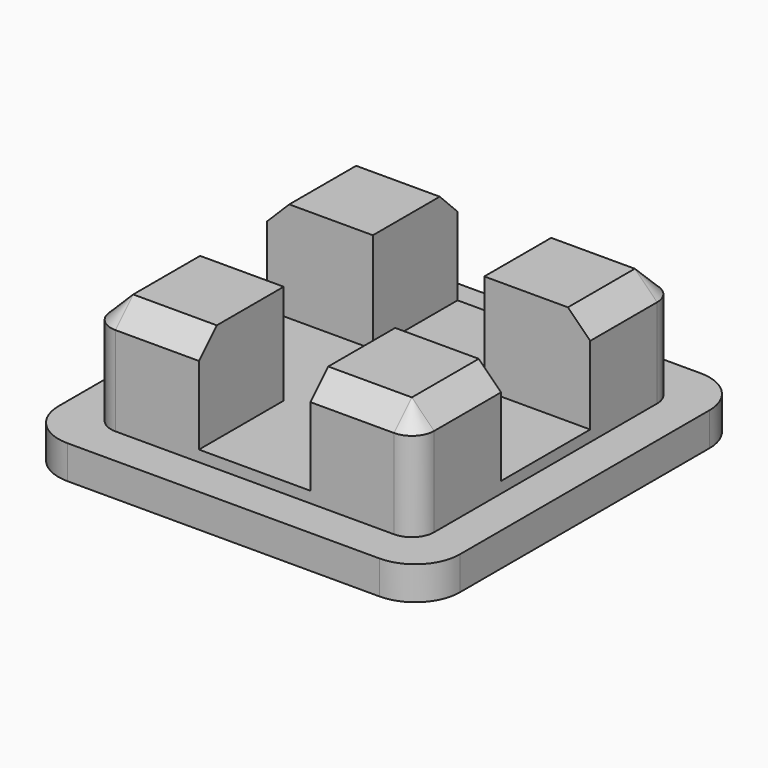
from build123d import *

# Parameters (mm, degrees)
F1_DEPTH = 3
F3_DEPTH = 10
F5_DEPTH = 9
F6_SIZE  = 1.99999


# Not quite as in the source:
# - a fillet or chamfer is up to 0.001 mm smaller than in the source, because OpenCascade refuses the exact size


with BuildPart() as f1:
    # F0 (on Top) → F1 (new body)
    with BuildSketch(Plane.XY):
        with BuildLine():
            Line((16.3916659281, 18.4843443355), (-11.6083340719, 18.4843443355))
            ThreePointArc((-11.6083340719, 18.4843443355), (-14.4367611967, 17.3127714603), (-15.6083340719, 14.4843443355))
            Line((-15.6083340719, 14.4843443355), (-15.6083340719, -13.5156556645))
            ThreePointArc((-15.6083340719, -13.5156556645), (-14.4367611967, -16.3440827892), (-11.6083340719, -17.5156556645))
            Line((-11.6083340719, -17.5156556645), (16.3916659281, -17.5156556645))
            ThreePointArc((16.3916659281, -17.5156556645), (19.2200930528, -16.3440827892), (20.3916659281, -13.5156556645))
            Line((20.3916659281, -13.5156556645), (20.3916659281, 14.4843443355))
            ThreePointArc((20.3916659281, 14.4843443355), (19.2200930528, 17.3127714603), (16.3916659281, 18.4843443355))
        make_face()
    extrude(amount=F1_DEPTH)

    # F2 (on face) → F3 (join)
    with BuildSketch(Plane.XY.offset(3)):
        with BuildLine():
            Line((14.8916659281, 14.9843443355), (-10.1083340719, 14.9843443355))
            ThreePointArc((-10.1083340719, 14.9843443355), (-11.5225476343, 14.3985578979), (-12.1083340719, 12.9843443355))
            Line((-12.1083340719, 12.9843443355), (-12.1083340719, -12.0156556645))
            ThreePointArc((-12.1083340719, -12.0156556645), (-11.5225476343, -13.4298692268), (-10.1083340719, -14.0156556645))
            Line((-10.1083340719, -14.0156556645), (14.8916659281, -14.0156556645))
            ThreePointArc((14.8916659281, -14.0156556645), (16.3058794904, -13.4298692268), (16.8916659281, -12.0156556645))
            Line((16.8916659281, -12.0156556645), (16.8916659281, 12.9843443355))
            ThreePointArc((16.8916659281, 12.9843443355), (16.3058794904, 14.3985578979), (14.8916659281, 14.9843443355))
        make_face()
    extrude(amount=F3_DEPTH)

    # F4 (on face) → F5 (cut)
    with BuildSketch(Plane.XY.offset(13)):
        Polygon((7.3916660622, 14.9843443355), (-2.6083340719, 14.9843443355), (-2.6083340719, 5.4843444377), (-12.1083340719, 5.4843444377), (-12.1083340719, -4.5156556645), (-2.6083340719, -4.5156556645), (-2.6083340719, -14.0156556645), (7.3916660622, -14.0156556645), (7.3916660622, -4.5156556645), (16.8916659281, -4.5156556645), (16.8916659281, 5.4843444377), (7.3916660622, 5.4843444377), align=None)
    extrude(amount=-F5_DEPTH, mode=Mode.SUBTRACT)

    # F6 (size 2 in the source; OpenCascade refuses exactly that, so slightly less here)
    f6_edges = [f1.edges().sort_by_distance(p)[0] for p in [
        (11.141666, -14.015656, 13),
        (-6.358334, -14.015656, 13),
        (16.891666, 9.234344, 13),
        (-12.108334, 9.234344, 13),
    ]]
    chamfer(f6_edges, length=F6_SIZE)


solid = f1.part
